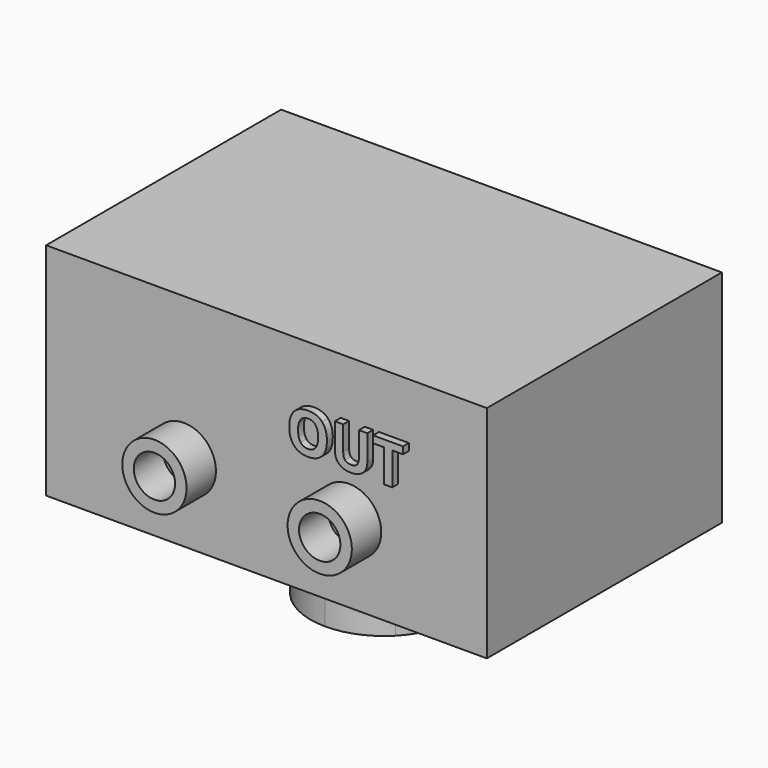
from build123d import *

# Parameters (mm, degrees)
F1_DEPTH  = 152.4
F2_DEPTH  = 50.8
F4_DEPTH  = 25.4
F5_W      = 100.7168591022
F5_H      = 42.3558056355
F6_DEPTH  = 6.35
F7_SIZE   = 2.54
F10_DEPTH = 5.08


with BuildPart() as f1:
    # F0 (on Top) → F1 (new body)
    with BuildSketch(Plane.XY):
        with BuildLine():
            Line((152.4, 0), (50.8, 0))
            ThreePointArc((50.8, 0), (47.0438920676, -19.1706082098), (36.3310149947, -35.5063001375))
            ThreePointArc((36.3310149947, -35.5063001375), (19.7093880297, -46.820722159), (0, -50.8))
            Line((0, -50.8), (0, -101.6))
            Line((0, -101.6), (152.4, -101.6))
            Line((152.4, -101.6), (152.4, 0))
        make_face()
        with BuildLine():
            ThreePointArc((0, 50.8), (35.9210244843, 35.9210244843), (50.8, 0))
            Line((50.8, 0), (152.4, 0))
            Line((152.4, 0), (152.4, 101.6))
            Line((152.4, 101.6), (0, 101.6))
            Line((0, 101.6), (0, 50.8))
        make_face()
        with BuildLine():
            ThreePointArc((0, -50.8), (-50.8, 0), (0, 50.8))
            Line((0, 50.8), (0, 101.6))
            Line((0, 101.6), (-152.4, 101.6))
            Line((-152.4, 101.6), (-152.4, -101.6))
            Line((-152.4, -101.6), (0, -101.6))
            Line((0, -101.6), (0, -50.8))
        make_face()
        with BuildLine():
            Line((0, -50.8), (0, 0))
            Line((0, 0), (0, 50.8))
            ThreePointArc((0, 50.8), (-50.8, 0), (0, -50.8))
        make_face()
        with BuildLine():
            Line((0, 50.8), (0, 0))
            Line((0, 0), (50.8, 0))
            ThreePointArc((50.8, 0), (35.9210244843, 35.9210244843), (0, 50.8))
        make_face()
        with BuildLine():
            Line((36.3310149947, -35.5063001375), (0, 0))
            Line((0, 0), (0, -50.8))
            ThreePointArc((0, -50.8), (19.7093880297, -46.820722159), (36.3310149947, -35.5063001375))
        make_face()
        with BuildLine():
            Line((50.8, 0), (0, 0))
            Line((0, 0), (36.3310149947, -35.5063001375))
            ThreePointArc((36.3310149947, -35.5063001375), (47.0438920676, -19.1706082098), (50.8, 0))
        make_face()
    extrude(amount=F1_DEPTH)

    # F0 (on Top) → F2 (join)
    with BuildSketch(Plane.XY):
        with BuildLine():
            Line((36.3310149947, -35.5063001375), (0, 0))
            Line((0, 0), (0, -50.8))
            ThreePointArc((0, -50.8), (19.7093880297, -46.820722159), (36.3310149947, -35.5063001375))
        make_face()
        with BuildLine():
            Line((50.8, 0), (0, 0))
            Line((0, 0), (36.3310149947, -35.5063001375))
            ThreePointArc((36.3310149947, -35.5063001375), (47.0438920676, -19.1706082098), (50.8, 0))
        make_face()
        with BuildLine():
            Line((0, 50.8), (0, 0))
            Line((0, 0), (50.8, 0))
            ThreePointArc((50.8, 0), (35.9210244843, 35.9210244843), (0, 50.8))
        make_face()
        with BuildLine():
            Line((0, -50.8), (0, 0))
            Line((0, 0), (0, 50.8))
            ThreePointArc((0, 50.8), (-50.8, 0), (0, -50.8))
        make_face()
    extrude(amount=-F2_DEPTH)

    # F3 (on face) → F4 (join)
    with BuildSketch(Plane.XZ.offset(101.6)):
        with BuildLine():
            ThreePointArc((34.925, 53.1082823873), (57.15, 30.8832823873), (79.375, 53.1082823873))
            Line((79.375, 53.1082823873), (71.4375, 53.1082823873))
            ThreePointArc((71.4375, 53.1082823873), (57.15, 38.8207823873), (42.8625, 53.1082823873))
            Line((42.8625, 53.1082823873), (34.925, 53.1082823873))
        make_face()
        with BuildLine():
            Line((71.4375, 53.1082823873), (79.375, 53.1082823873))
            ThreePointArc((79.375, 53.1082823873), (57.15, 75.3332823873), (34.925, 53.1082823873))
            Line((34.925, 53.1082823873), (42.8625, 53.1082823873))
            ThreePointArc((42.8625, 53.1082823873), (57.15, 67.3957823873), (71.4375, 53.1082823873))
        make_face()
        with BuildLine():
            ThreePointArc((-34.925, 53.1082823873), (-57.15, 75.3332823873), (-79.375, 53.1082823873))
            Line((-79.375, 53.1082823873), (-71.4375, 53.1082823873))
            ThreePointArc((-71.4375, 53.1082823873), (-57.15, 67.3957823873), (-42.8625, 53.1082823873))
            Line((-42.8625, 53.1082823873), (-34.925, 53.1082823873))
        make_face()
        with BuildLine():
            Line((-71.4375, 53.1082823873), (-79.375, 53.1082823873))
            ThreePointArc((-79.375, 53.1082823873), (-57.15, 30.8832823873), (-34.925, 53.1082823873))
            Line((-34.925, 53.1082823873), (-42.8625, 53.1082823873))
            ThreePointArc((-42.8625, 53.1082823873), (-57.15, 38.8207823873), (-71.4375, 53.1082823873))
        make_face()
    extrude(amount=F4_DEPTH)

    # F9 (on face) + F8 (on face) → F10 (join)
    with BuildSketch(Plane.XZ.offset(101.6)):
        Polygon((91.0699902064, 86.2468481064), (91.0699902064, 108.7812007722), (98.4956073484, 108.7812007722), (98.4956073484, 113.6078519145), (77.8356241709, 113.6078519145), (77.8356241709, 108.7812007722), (85.2672297139, 108.7812007722), (85.2672297139, 86.2468481064), align=None)
        with BuildLine():
            Line((73.811418752, 113.6078519145), (68.0266234623, 113.6078519145))
            Line((68.0266234623, 113.6078519145), (68.0266234623, 96.894224944))
            add(Edge.make_bspline(
                [(66.7451056652, 92.226266426), (68.0266234623, 93.7143840549), (68.0266234623, 96.894224944)],
                knots=[0, 0, 0, 1, 1, 1], degree=2))
            add(Edge.make_bspline(
                [(62.6190974306, 90.7381487971), (65.4635878681, 90.7381487971), (66.7451056652, 92.226266426)],
                knots=[0, 0, 0, 1, 1, 1], degree=2))
            add(Edge.make_bspline(
                [(58.4062573827, 92.2172838246), (59.6787925784, 90.7381487971), (62.6190974306, 90.7381487971)],
                knots=[0, 0, 0, 1, 1, 1], degree=2))
            add(Edge.make_bspline(
                [(57.1337221869, 96.8582945384), (57.1337221869, 93.6964188521), (58.4062573827, 92.2172838246)],
                knots=[0, 0, 0, 1, 1, 1], degree=2))
            Line((57.1337221869, 96.8582945384), (57.1337221869, 113.6078519145))
            Line((57.1337221869, 113.6078519145), (51.3549152982, 113.6078519145))
            Line((51.3549152982, 113.6078519145), (51.3549152982, 95.977999603))
            add(Edge.make_bspline(
                [(54.2742607472, 88.5763360647), (51.3549152982, 91.283093281), (51.3549152982, 95.977999603)],
                knots=[0, 0, 0, 1, 1, 1], degree=2))
            add(Edge.make_bspline(
                [(62.4693874076, 85.8695788484), (57.1936061962, 85.8695788484), (54.2742607472, 88.5763360647)],
                knots=[0, 0, 0, 1, 1, 1], degree=2))
            add(Edge.make_bspline(
                [(68.5326433401, 87.0882184358), (65.9666135454, 85.8695788484), (62.4693874076, 85.8695788484)],
                knots=[0, 0, 0, 1, 1, 1], degree=2))
            add(Edge.make_bspline(
                [(72.4550459434, 90.5884387741), (71.0986731348, 88.3068580232), (68.5326433401, 87.0882184358)],
                knots=[0, 0, 0, 1, 1, 1], degree=2))
            add(Edge.make_bspline(
                [(73.811418752, 95.906138792), (73.811418752, 92.870019525), (72.4550459434, 90.5884387741)],
                knots=[0, 0, 0, 1, 1, 1], degree=2))
            Line((73.811418752, 95.906138792), (73.811418752, 113.6078519145))
        make_face()
    with BuildSketch(Plane.XZ.offset(101.6)):
        with BuildLine():
            add(Edge.make_bspline(
                [(45.8695400545, 99.9662746164), (45.8695400545, 93.1694395711), (42.5010645364, 89.5195092097)],
                knots=[0, 0, 0, 1, 1, 1], degree=2))
            add(Edge.make_bspline(
                [(42.5280123406, 110.4070516222), (45.8695400545, 106.7750864636), (45.8695400545, 99.9662746164)],
                knots=[0, 0, 0, 1, 1, 1], degree=2))
            add(Edge.make_bspline(
                [(32.8806984568, 114.0390167808), (39.1864846266, 114.0390167808), (42.5280123406, 110.4070516222)],
                knots=[0, 0, 0, 1, 1, 1], degree=2))
            add(Edge.make_bspline(
                [(23.1974541675, 110.4369936268), (26.574912287, 114.0390167808), (32.8806984568, 114.0390167808)],
                knots=[0, 0, 0, 1, 1, 1], degree=2))
            add(Edge.make_bspline(
                [(19.8199960481, 100.002205022), (19.8199960481, 106.8349704728), (23.1974541675, 110.4369936268)],
                knots=[0, 0, 0, 1, 1, 1], degree=2))
            add(Edge.make_bspline(
                [(23.1884715661, 89.5195092097), (19.8199960481, 93.1694395711), (19.8199960481, 100.002205022)],
                knots=[0, 0, 0, 1, 1, 1], degree=2))
            add(Edge.make_bspline(
                [(32.8447680513, 85.8695788484), (26.5569470842, 85.8695788484), (23.1884715661, 89.5195092097)],
                knots=[0, 0, 0, 1, 1, 1], degree=2))
            add(Edge.make_bspline(
                [(42.5010645364, 89.5195092097), (39.1325890184, 85.8695788484), (32.8447680513, 85.8695788484)],
                knots=[0, 0, 0, 1, 1, 1], degree=2))
        make_face()
        with BuildLine():
            add(Edge.make_bspline(
                [(25.9042113838, 99.9662746164), (25.9042113838, 95.3791595109), (27.6438418514, 93.058654154)],
                knots=[0, 0, 0, 1, 1, 1], degree=2))
            add(Edge.make_bspline(
                [(27.6618070541, 106.8768892793), (25.9042113838, 104.547401321), (25.9042113838, 99.9662746164)],
                knots=[0, 0, 0, 1, 1, 1], degree=2))
            add(Edge.make_bspline(
                [(32.8806984568, 109.2063772376), (29.4194027245, 109.2063772376), (27.6618070541, 106.8768892793)],
                knots=[0, 0, 0, 1, 1, 1], degree=2))
            add(Edge.make_bspline(
                [(39.7853247188, 99.9662746164), (39.7853247188, 109.2063772376), (32.8806984568, 109.2063772376)],
                knots=[0, 0, 0, 1, 1, 1], degree=2))
            add(Edge.make_bspline(
                [(32.8447680513, 90.7381487971), (39.7853247188, 90.7381487971), (39.7853247188, 99.9662746164)],
                knots=[0, 0, 0, 1, 1, 1], degree=2))
            add(Edge.make_bspline(
                [(27.6438418514, 93.058654154), (29.3834723189, 90.7381487971), (32.8447680513, 90.7381487971)],
                knots=[0, 0, 0, 1, 1, 1], degree=2))
        make_face(mode=Mode.SUBTRACT)
    extrude(amount=F10_DEPTH)


with BuildPart() as f6:
    # F5 (on face) → F6 (new body)
    with BuildSketch(Plane(origin=(0, 101.6, 0), x_dir=(-1, 0, 0), z_dir=(0, 1, 0))):
        with Locations((66.9497698545, 98.8216623664)):
            Rectangle(F5_W, F5_H)
    extrude(amount=F6_DEPTH)

    # F7
    f7_edges = [f6.edges().sort_by_distance(p)[0] for p in [
        (-66.94977, 107.95, 119.999565),
        (-117.308199, 107.95, 98.821662),
        (-16.59134, 107.95, 98.821662),
        (-66.94977, 107.95, 77.64376),
    ]]
    chamfer(f7_edges, length=F7_SIZE)


solid = Compound([f1.part, f6.part])
